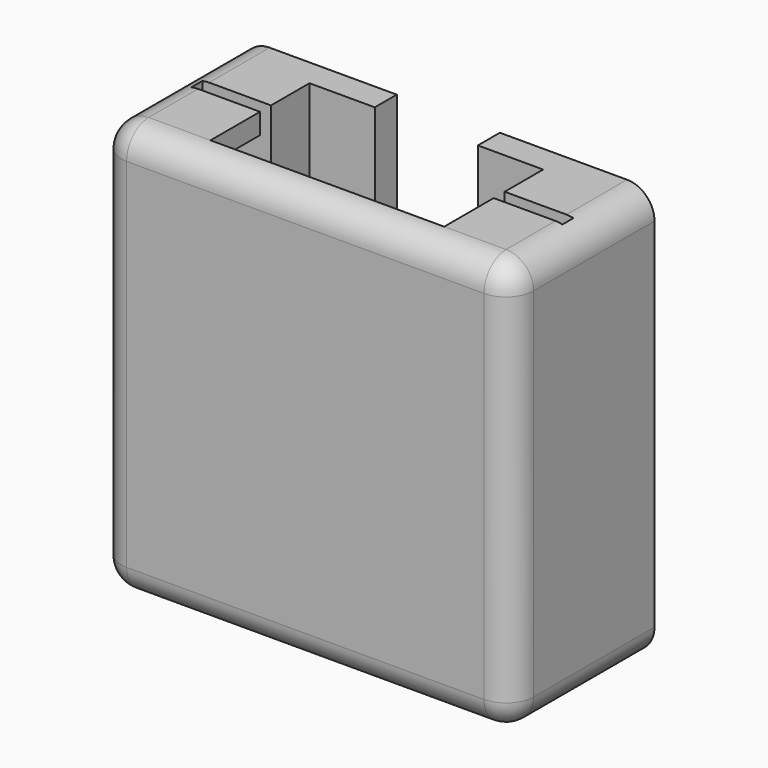
from build123d import *

# Parameters (mm, degrees)
F0_W         = 5
F0_H         = 27
F0_W_2       = 4.75
F0_H_2       = 1.5
F1_DEPTH     = 2
F2_DEPTH     = 5.5
F3_DEPTH     = 11
F5_DEPTH     = 28.5
F4_W         = 17
F4_H         = 3
F6_DEPTH     = 1.5
F7_W         = 30
F7_H         = 30
F7_W_2       = 27
F7_H_2       = 27
F7_W_3       = 23
F7_H_3       = 23
F8_DEPTH     = 2
F9_DEPTH     = 1.5
F10_T1_DEPTH = 21
F10_2_F1_R   = 2
F10_2_F2_R   = 2
F10_2_F3_R   = 1.9999
F10_2_F4_R   = 1.9999


# Not quite as in the source:
# - a fillet or chamfer that OpenCascade refuses, or shapes differently, is made with other operations: its cross-section is extruded or revolved along the edge and cut away or added
# - a fillet or chamfer is up to 0.001 mm smaller than in the source, because OpenCascade refuses the exact size


with BuildPart() as f1:
    # F0 (on Front) → F1 (new body)
    with BuildSketch(Plane.XZ):
        with Locations((11, 0)):
            Rectangle(F0_W, F0_H)
        with BuildLine():
            Line((-8.5, -13.5), (8.5, -13.5))
            Line((8.5, -13.5), (8.5, 13.5))
            Line((8.5, 13.5), (3.75, 13.5))
            Line((3.75, 13.5), (3.75, -3.038))
            ThreePointArc((3.75, -3.038), (0, -6.788), (-3.75, -3.038))
            Line((-3.75, -3.038), (-3.75, 13.5))
            Line((-3.75, 13.5), (-8.5, 13.5))
            Line((-8.5, 13.5), (-8.5, -13.5))
        make_face()
        with Locations((-11, 0)):
            Rectangle(F0_W, F0_H)
        Polygon((13.5, 13.5), (13.5, -13.5), (8.5, -13.5), (-8.5, -13.5), (-13.5, -13.5), (-13.5, 13.5), (-8.5, 13.5), (-8.5, 15), (-15, 15), (-15, -15), (15, -15), (15, 15), (8.5, 15), (8.5, 13.5), align=None)
        with Locations((-6.125, 14.25)):
            Rectangle(F0_W_2, F0_H_2)
        with Locations((6.125, 14.25)):
            Rectangle(F0_W_2, F0_H_2)
    extrude(amount=F1_DEPTH)

    # F0 (on Front) → F2 (join)
    with BuildSketch(Plane.XZ):
        with Locations((-11, 0)):
            Rectangle(F0_W, F0_H)
        with Locations((11, 0)):
            Rectangle(F0_W, F0_H)
        Polygon((13.5, 13.5), (13.5, -13.5), (8.5, -13.5), (-8.5, -13.5), (-13.5, -13.5), (-13.5, 13.5), (-8.5, 13.5), (-8.5, 15), (-15, 15), (-15, -15), (15, -15), (15, 15), (8.5, 15), (8.5, 13.5), align=None)
    extrude(amount=F2_DEPTH)

    # F0 (on Front) → F3 (join)
    with BuildSketch(Plane.XZ):
        Polygon((13.5, 13.5), (13.5, -13.5), (8.5, -13.5), (-8.5, -13.5), (-13.5, -13.5), (-13.5, 13.5), (-8.5, 13.5), (-8.5, 15), (-15, 15), (-15, -15), (15, -15), (15, 15), (8.5, 15), (8.5, 13.5), align=None)
    extrude(amount=F3_DEPTH)

    # F4 (on face) → F5 (cut, through all)
    with BuildSketch(Plane.XY.offset(-13.5)):
        Polygon((-13.5, -5.5), (-13.5, -6.5), (-8.5, -6.5), (8.5, -6.5), (13.5, -6.5), (13.5, -5.5), (8.5, -5.5), (-8.5, -5.5), align=None)
    extrude(amount=F5_DEPTH, mode=Mode.SUBTRACT)

    # F4 (on face) → F6 (cut, through all)
    with BuildSketch(Plane.XY.offset(-13.5)):
        with Locations((0, -8)):
            Rectangle(F4_W, F4_H)
    extrude(amount=-F6_DEPTH, mode=Mode.SUBTRACT)

    # F10: fillet of radius 2 on 4 edges, made by hand

    # F10_s2 → F10_t1 (cut)
    with BuildSketch(Plane.XZ.offset(-5)):
        with BuildLine():
            ThreePointArc((13, -15), (14.4142135624, -14.4142135624), (15, -13))
            Line((15, -13), (15, -15))
            Line((15, -15), (13, -15))
        make_face()
        with BuildLine():
            ThreePointArc((13, 15), (14.4142135624, 14.4142135624), (15, 13))
            Line((15, 13), (15, 15))
            Line((15, 15), (13, 15))
        make_face()
        with BuildLine():
            ThreePointArc((-13, 15), (-14.4142135624, 14.4142135624), (-15, 13))
            Line((-15, 13), (-15, 15))
            Line((-15, 15), (-13, 15))
        make_face()
        with BuildLine():
            ThreePointArc((-15, -13), (-14.4142135624, -14.4142135624), (-13, -15))
            Line((-13, -15), (-15, -15))
            Line((-15, -15), (-15, -13))
        make_face()
    extrude(amount=F10_T1_DEPTH, mode=Mode.SUBTRACT)


with BuildPart() as f8:
    # F7 (on face) → F8 (new body)
    with BuildSketch(Plane.XZ.offset(11)):
        Rectangle(F7_W, F7_H)
        Rectangle(F7_W_2, F7_H_2, mode=Mode.SUBTRACT)
        Polygon((13.5, 13.5), (8.5, 13.5), (-8.5, 13.5), (-13.5, 13.5), (-13.5, -13.5), (13.5, -13.5), align=None)
        Rectangle(F7_W_3, F7_H_3, mode=Mode.SUBTRACT)
        Rectangle(F7_W_3, F7_H_3)
    extrude(amount=F8_DEPTH)

    # F7 (on face) → F9 (join)
    with BuildSketch(Plane.XZ.offset(11)):
        Polygon((13.5, 13.5), (8.5, 13.5), (-8.5, 13.5), (-13.5, 13.5), (-13.5, -13.5), (13.5, -13.5), align=None)
        Rectangle(F7_W_3, F7_H_3, mode=Mode.SUBTRACT)
    extrude(amount=-F9_DEPTH)

    # F10#2: fillet of radius 2 on 8 edges, made by hand

    # F10_2_f1
    f10_2_f1_edges = [f8.edges().sort_by_distance(p)[0] for p in [
        (-15, -12, -15),
    ]]
    fillet(f10_2_f1_edges, radius=F10_2_F1_R)

    # F10_2_f2
    f10_2_f2_edges = [f8.edges().sort_by_distance(p)[0] for p in [
        (15, -12, -15),
    ]]
    fillet(f10_2_f2_edges, radius=F10_2_F2_R)

    # F10_2_f3 (radius 2 in the source; OpenCascade refuses exactly that, so slightly less here)
    f10_2_f3_edges = [f8.edges().sort_by_distance(p)[0] for p in [
        (0, -13, -15),
    ]]
    fillet(f10_2_f3_edges, radius=F10_2_F3_R)

    # F10_2_f4 (radius 2 in the source; OpenCascade refuses exactly that, so slightly less here)
    f10_2_f4_edges = [f8.edges().sort_by_distance(p)[0] for p in [
        (-15, -11.00005, 15),
    ]]
    fillet(f10_2_f4_edges, radius=F10_2_F4_R)


solid = Compound([f1.part, f8.part])
